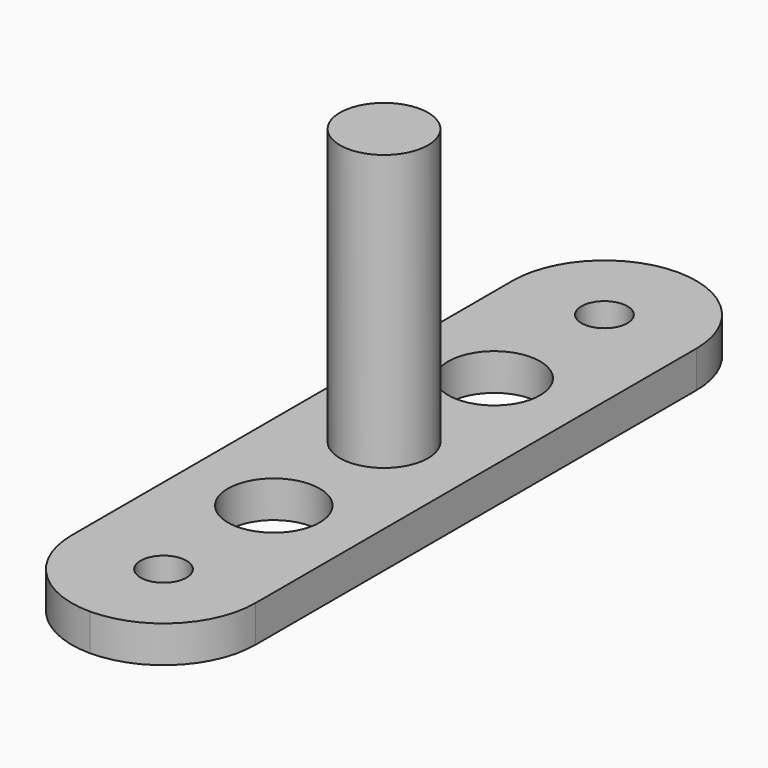
from build123d import *

# Parameters (mm, degrees)
F0_R     = 3.048
F1_DEPTH = 9.525
F2_W     = 12.7
F2_H     = 50.8
F3_DEPTH = 2.54
F4_R     = 6.34999
F5_R     = 1.5875
F5_R_2   = 3.175
F6_DEPTH = 2.541


# Not quite as in the source:
# - a fillet or chamfer is up to 0.001 mm smaller than in the source, because OpenCascade refuses the exact size


with BuildPart() as f1:
    # F0 (on Top) → F1 (new body, symmetric)
    with BuildSketch(Plane.XY):
        Circle(F0_R)
    extrude(amount=F1_DEPTH, both=True)

    # F2 (on face) → F3 (join)
    with BuildSketch(Plane(origin=(0, 0, -9.525), x_dir=(1, 0, 0), z_dir=(0, 0, -1))):
        Rectangle(F2_W, F2_H)
    extrude(amount=F3_DEPTH)

    # F4 (radius 6.35 in the source; OpenCascade refuses exactly that, so slightly less here)
    f4_edges = [f1.edges().sort_by_distance(p)[0] for p in [
        (-6.35, 25.4, -10.795),
        (6.35, 25.4, -10.795),
        (-6.35, -25.4, -10.795),
        (6.35, -25.4, -10.795),
    ]]
    fillet(f4_edges, radius=F4_R)

    # F5 (on face) → F6 (cut, through all)
    with BuildSketch(Plane.XY.offset(-9.525)):
        with Locations((0, 19.05)):
            Circle(F5_R)
        with Locations((0, 9.525)):
            Circle(F5_R_2)
        with Locations((0, -19.05)):
            Circle(F5_R)
        with Locations((0, -9.525)):
            Circle(F5_R_2)
    extrude(amount=-F6_DEPTH, mode=Mode.SUBTRACT)


solid = f1.part
